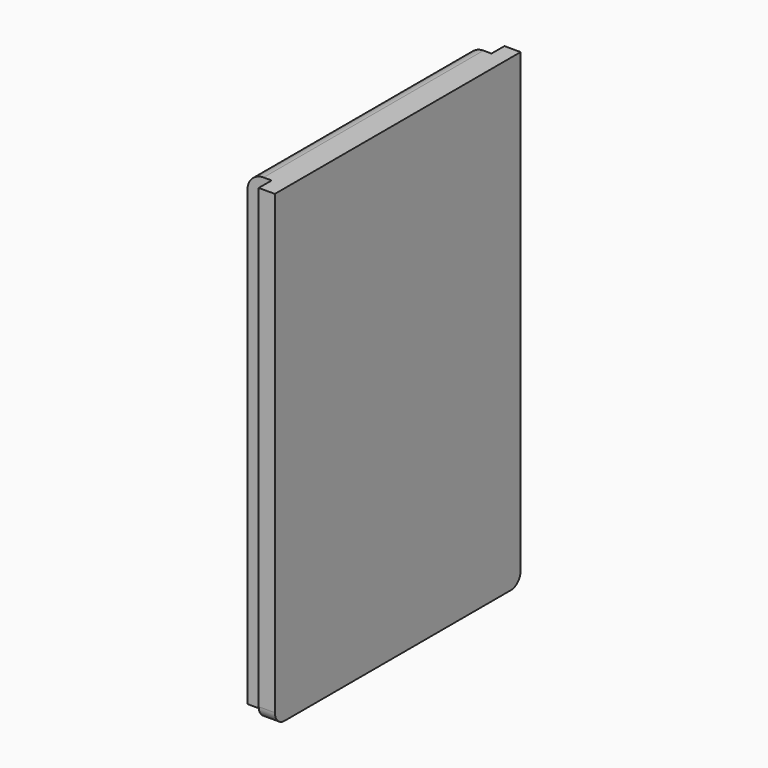
from build123d import *

# Parameters (mm, degrees)
F1_DEPTH     = 29.464
F2_W         = 12.192
F2_H         = 2.54
F3_DEPTH     = 1.27
F4_R         = 0.508
F5_R         = 1.016
F6_TEXT_SIZE = 5.2916666667
F7_DEPTH     = 0.508
F8_R         = 0.762


# Not quite as in the source:
# - Text() gives the source's letters only with a copy of the font that has no kerning and outlines rounded to 1/6400 em; it was checked with that copy


with BuildPart() as f1:
    # F0 (on Top) → F1 (new body)
    with BuildSketch(Plane.XY):
        Polygon((11.5668522194, 3.8801730177), (10.0428522194, 3.8801730177), (10.0428522194, -13.3918269823), (11.5668522194, -13.3918269823), (11.5668522194, -14.4078269823), (12.5828522194, -14.4078269823), (12.5828522194, -13.3918269823), (12.5828522194, 3.8801730177), (12.5828522194, 4.8961730177), (11.5668522194, 4.8961730177), align=None)
    extrude(amount=F1_DEPTH)

    # F2 (on face) → F3 (cut)
    with BuildSketch(Plane(origin=(10.0428522194, 0, 0), x_dir=(0, -1, 0), z_dir=(-1, 0, 0))):
        with Locations((4.7558269823, 25.654)):
            Rectangle(F2_W, F2_H)
    extrude(amount=-F3_DEPTH, mode=Mode.SUBTRACT)

    # F4
    f4_edges = [f1.edges().sort_by_distance(p)[0] for p in [
        (11.312852, -4.755827, 26.924),
        (11.312852, 1.340173, 25.654),
        (11.312852, -4.755827, 24.384),
        (11.312852, -10.851827, 25.654),
    ]]
    fillet(f4_edges, radius=F4_R)

    # F5
    f5_edges = [f1.edges().sort_by_distance(p)[0] for p in [
        (10.042852, -4.755827, 29.464),
    ]]
    fillet(f5_edges, radius=F5_R)

    # F6 (on face) → F7 (join)
    with BuildSketch(Plane(origin=(10.0428522194, 0, 0), x_dir=(0, -1, 0), z_dir=(-1, 0, 0))):
        with Locations((1.3546909146, 1.650901337)):
            Text('9V', F6_TEXT_SIZE, font='Open Sans', font_style=FontStyle.BOLD, text_align=(TextAlign.LEFT, TextAlign.BOTTOM))
    extrude(amount=F7_DEPTH)

    # F8
    f8_edges = [f1.edges().sort_by_distance(p)[0] for p in [
        (12.074852, 4.896173, 0),
        (12.074852, -14.407827, 0),
    ]]
    fillet(f8_edges, radius=F8_R)


solid = f1.part
